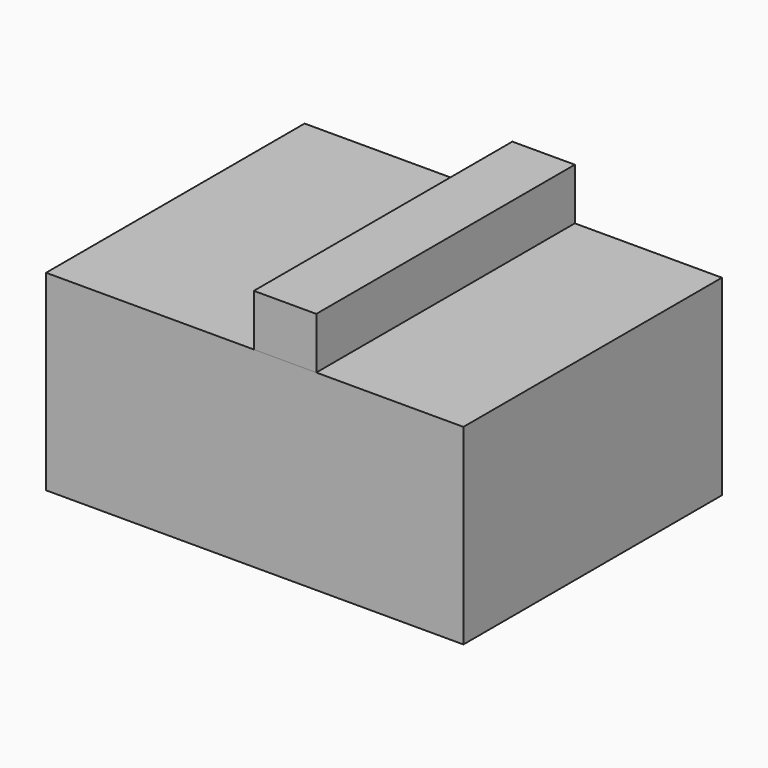
from build123d import *

# Parameters (mm, degrees)
F0_W     = 65.3258264065
F0_H     = 60.2281540632
F1_DEPTH = 101.6
F0_W_2   = 19.6354985237
F0_H_2   = 16.2370502949
F2_W     = 101.6
F2_H     = 60.2281540632
F3_DEPTH = 131.2111467123


with BuildPart() as f1:
    # F0 (on Front) → F1 (new body)
    with BuildSketch(Plane.XZ):
        with Locations((32.6629132032, 30.1140770316)):
            Rectangle(F0_W, F0_H)
    extrude(amount=F1_DEPTH)


with BuildPart() as f1b:
    # F0 (on Front) → F1, piece 2 (new body)
    with BuildSketch(Plane.XZ):
        with Locations((75.1435756683, 68.3466792107)):
            Rectangle(F0_W_2, F0_H_2)
    extrude(amount=F1_DEPTH)


with BuildPart() as f3:
    # F2 (on face) → F3 (new body)
    with BuildSketch(Plane(origin=(0, 0, 0), x_dir=(0, -1, 0), z_dir=(-1, 0, 0))):
        with Locations((50.8, 30.1140770316)):
            Rectangle(F2_W, F2_H)
    extrude(amount=-F3_DEPTH)


solid = Compound([f1.part, f1b.part, f3.part])
